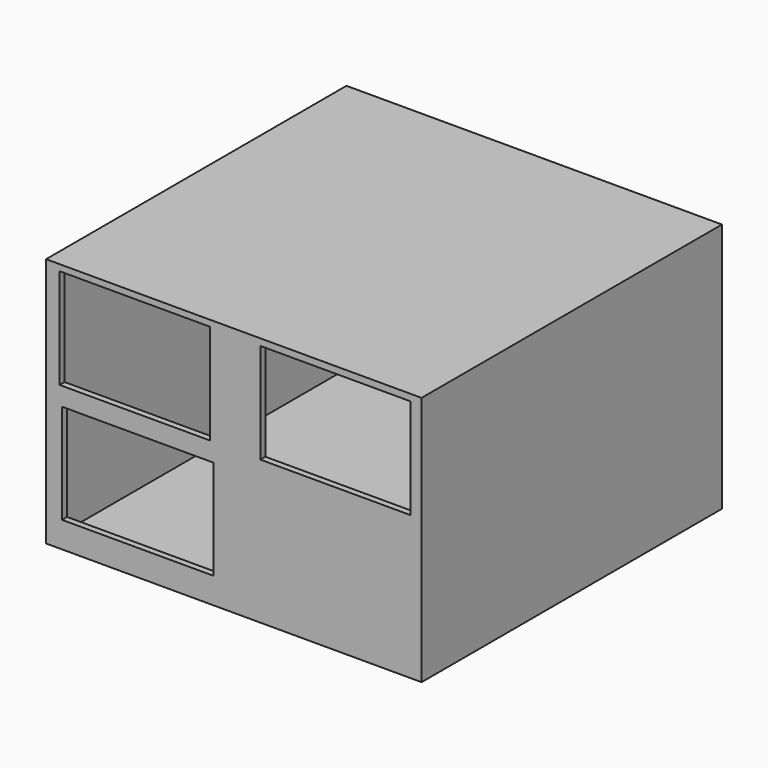
from build123d import *

# Parameters (mm, degrees)
F0_W     = 150
F0_H     = 100
F1_DEPTH = 150
F2_T     = -2.5
F3_W     = 60
F3_H     = 40
F4_DEPTH = 468.9
F5_W     = 60
F5_H     = 40
F6_DEPTH = 145
F7_W     = 60.590963345
F7_H     = 39.7856272757
F8_DEPTH = 146.1


# Not quite as in the source:
# - a feature names something its author has since deleted; it is built from what else it names


with BuildPart() as f1:
    # F0 (on Right) → F1 (new body)
    with BuildSketch(Plane.YZ):
        with Locations((-13.7818545103, -23.5450232641)):
            Rectangle(F0_W, F0_H)
    extrude(amount=F1_DEPTH)

    # F2 (hollow: no face is removed)
    offset(amount=F2_T, mode=Mode.SUBTRACT)

    # F3 (on Front) → F4 (cut)
    with BuildSketch(Plane.XZ):
        with Locations((35.4225549102, 3.9785955846)):
            Rectangle(F3_W, F3_H)
    extrude(amount=F4_DEPTH, mode=Mode.SUBTRACT)

    # F5 (on face) → F6 (cut)
    with BuildSketch(Plane.XZ.offset(88.7818545103)):
        with Locations((115.576479584, 3.7956100403)):
            Rectangle(F5_W, F5_H)
    extrude(amount=-F6_DEPTH, mode=Mode.SUBTRACT)

    # F7 (on face) → F8 (cut)
    with BuildSketch(Plane.XZ.offset(88.7818545103)):
        with Locations((36.6743972991, -43.25533472)):
            Rectangle(F7_W, F7_H)
    extrude(amount=-F8_DEPTH, mode=Mode.SUBTRACT)


solid = f1.part
